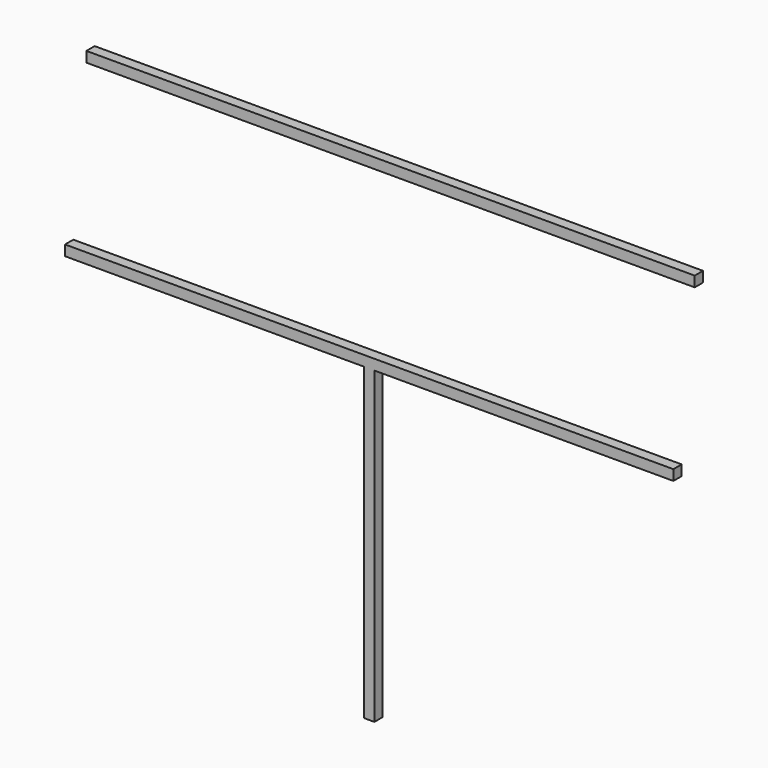
from build123d import *

# Parameters (mm, degrees)
F1_DEPTH = 33
F0_W     = 1934
F0_H     = 33


# Not quite as in the source:
# - a feature names something its author has since deleted; it is built from what else it names


with BuildPart() as f1:
    # F0 (on Front) → F1 (new body)
    with BuildSketch(Plane.XZ):
        Polygon((983.5, 983.5), (983.5, 0), (1016.5, 0), (1016.5, 983.5), (1967, 983.5), (1967, 1016.5), (33, 1016.5), (33, 983.5), align=None)
    extrude(amount=F1_DEPTH)


with BuildPart() as f1b:
    # F0 (on Front) → F1, piece 2 (new body)
    with BuildSketch(Plane.XZ):
        with Locations((1067.8651331067, 1563.7987890244)):
            Rectangle(F0_W, F0_H)
    extrude(amount=F1_DEPTH)


solid = Compound([f1.part, f1b.part])
